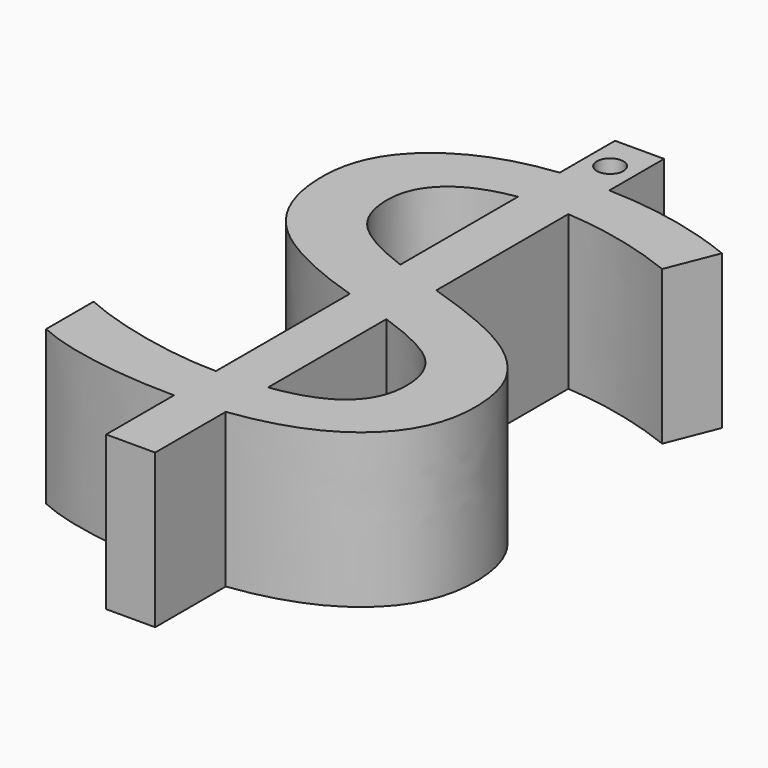
from build123d import *

# Parameters (mm, degrees)
F0_TEXT_SIZE = 126.5822806292
F1_DEPTH     = 25
F2_R         = 2.1554604173
F3_DEPTH     = 25


# Not quite as in the source:
# - Text() gives the source's letters only with a copy of the font that has no kerning and outlines rounded to 1/6400 em; it was checked with that copy


with BuildPart() as f1:
    # F0 (on Top) → F1 (new body)
    with BuildSketch(Plane.XY):
        with Locations((-40.5854433775, -50.4113920033)):
            Text('$', F0_TEXT_SIZE, font='Open Sans', text_align=(TextAlign.LEFT, TextAlign.BOTTOM))
    extrude(amount=F1_DEPTH)

    # F2 (on Top) → F3 (cut)
    with BuildSketch(Plane.XY):
        with Locations((-4.5651234686, 39.7870764136)):
            Circle(F2_R)
    extrude(amount=F3_DEPTH, mode=Mode.SUBTRACT)


solid = f1.part
